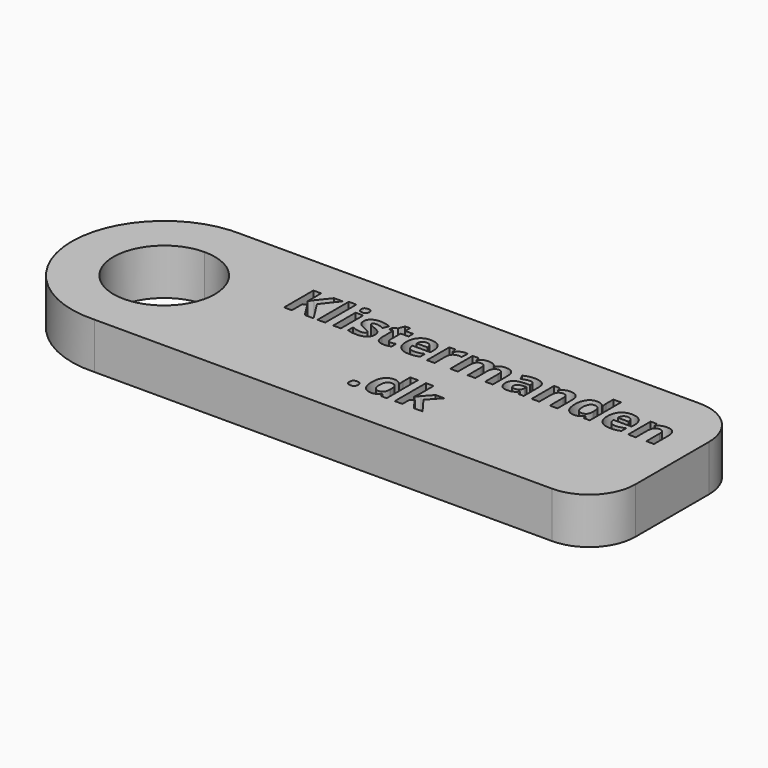
from build123d import *

# Parameters (mm, degrees)
F1_DEPTH     = 5
F2_TEXT_SIZE = 5.5555555556
F3_DEPTH     = 2


# Not quite as in the source:
# - Text() gives the source's letters only with a copy of the font that has no kerning and outlines rounded to 1/6400 em; it was checked with that copy


with BuildPart() as f1:
    # F0 (on Top) → F1 (new body)
    with BuildSketch(Plane.XY):
        with BuildLine():
            Line((-9.254835546, 30.4966073649), (-9.254835546, 34.9985063076))
            Line((-9.254835546, 34.9985063076), (-8.8090156204, 34.9985063076))
            ThreePointArc((-8.8090156204, 34.9985063076), (-19.254835546, 25.0084490208), (-8.8090156204, 15.018391734))
            Line((-8.8090156204, 15.018391734), (-9.254835546, 15.018391734))
            Line((-9.254835546, 15.018391734), (-9.254835546, 19.5202906767))
            ThreePointArc((-9.254835546, 19.5202906767), (-14.7429938901, 25.0084490208), (-9.254835546, 30.4966073649))
        make_face()
        with BuildLine():
            Line((-8.8090156204, 34.9985063076), (-9.254835546, 34.9985063076))
            Line((-9.254835546, 34.9985063076), (-9.254835546, 30.4966073649))
            ThreePointArc((-9.254835546, 30.4966073649), (-5.3741215647, 28.8891630021), (-3.7666772019, 25.0084490208))
            ThreePointArc((-3.7666772019, 25.0084490208), (-5.3741215647, 21.1277350394), (-9.254835546, 19.5202906767))
            Line((-9.254835546, 19.5202906767), (-9.254835546, 15.018391734))
            Line((-9.254835546, 15.018391734), (-8.8090156204, 15.018391734))
            ThreePointArc((-8.8090156204, 15.018391734), (-2.0278652522, 18.0967994078), (0.745164454, 25.0084490208))
            ThreePointArc((0.745164454, 25.0084490208), (-2.0278652522, 31.9200986337), (-8.8090156204, 34.9985063076))
        make_face()
        with BuildLine():
            Line((40.745164454, 34.9985063076), (-8.8090156204, 34.9985063076))
            ThreePointArc((-8.8090156204, 34.9985063076), (-2.0278652522, 31.9200986337), (0.745164454, 25.0084490208))
            ThreePointArc((0.745164454, 25.0084490208), (-2.0278652522, 18.0967994078), (-8.8090156204, 15.018391734))
            Line((-8.8090156204, 15.018391734), (40.745164454, 15.018391734))
            ThreePointArc((40.745164454, 15.018391734), (44.2806983599, 16.482857828), (45.745164454, 20.018391734))
            Line((45.745164454, 20.018391734), (45.745164454, 29.9985063076))
            ThreePointArc((45.745164454, 29.9985063076), (44.2806983599, 33.5340402135), (40.745164454, 34.9985063076))
        make_face()
    extrude(amount=-F1_DEPTH)

    # F2 (on Top) → F3 (cut)
    with BuildSketch(Plane.XY):
        with Locations((1.8102894206, 26.7789190232)):
            Text('Klistermanden', F2_TEXT_SIZE, font='Open Sans', font_style=FontStyle.BOLD, text_align=(TextAlign.LEFT, TextAlign.BOTTOM))
        with Locations((14.8024769206, 19.2233634677)):
            Text('.dk', F2_TEXT_SIZE, font='Open Sans', font_style=FontStyle.BOLD, text_align=(TextAlign.LEFT, TextAlign.BOTTOM))
    extrude(amount=-F3_DEPTH, mode=Mode.SUBTRACT)


solid = f1.part
